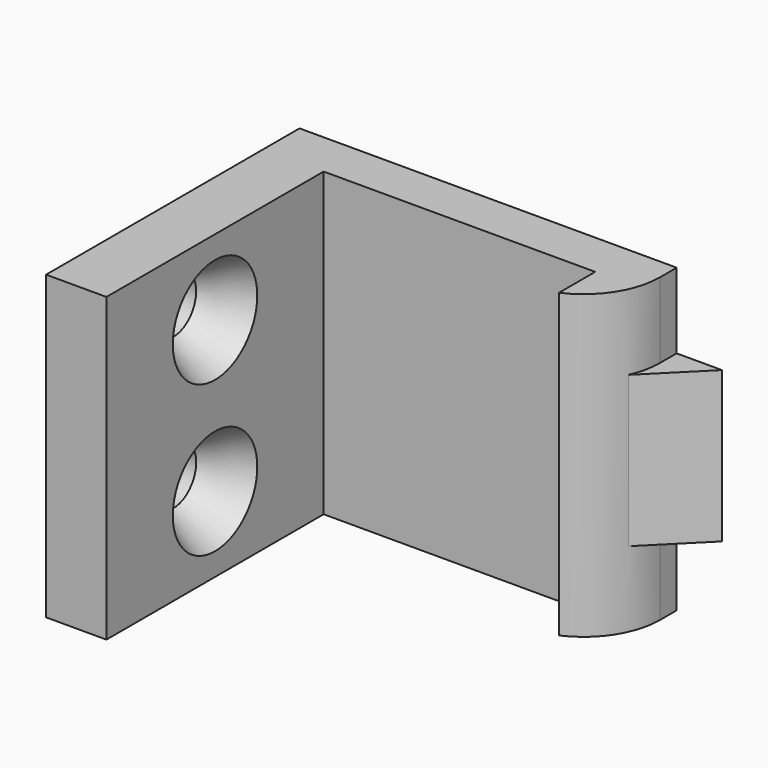
from build123d import *

# Parameters (mm, degrees)
F1_DEPTH       = 20
F2_DEPTH       = 15
F3_DEPTH       = 5
F5_D           = 3.8
F5_DEPTH       = 20
F5_CSINK_D     = 7
F5_CSINK_ANGLE = 60
F5_TIP         = 1.1416351762
F6_T4_DEPTH    = 43.1732604525
F6_T10_DEPTH   = 43.1732604525
F6_T16_DEPTH   = 43.1732604525
F6_T23_DEPTH   = 43.1732604525
F6_T29_DEPTH   = 43.1732604525


# Not quite as in the source:
# - a fillet or chamfer that OpenCascade refuses, or shapes differently, is made with other operations: its cross-section is extruded or revolved along the edge and cut away or added


with BuildPart() as f1:
    # F0 (on Top) → F1 (new body)
    with BuildSketch(Plane.XY):
        Polygon((-23.1947004795, 4.0139819533), (-23.1947004795, -16.9860180467), (-19.1947004795, -16.9860180467), (-19.1947004795, 1.0139819533), (-1.1947004795, 1.0139819533), (-1.1947004795, -1.9860180467), (1.8052995205, -1.9860180467), (1.8052995205, 1.0139819533), (1.8052995205, 4.0139819533), align=None)
    extrude(amount=F1_DEPTH)

    # F0 (on Top) → F2 (join)
    with BuildSketch(Plane.XY):
        Polygon((4.8052995205, 4.0139819533), (1.8052995205, 4.0139819533), (1.8052995205, 1.0139819533), align=None)
    extrude(amount=F2_DEPTH)

    # F0 (on Top) → F3 (cut)
    with BuildSketch(Plane.XY):
        Polygon((4.8052995205, 4.0139819533), (1.8052995205, 4.0139819533), (1.8052995205, 1.0139819533), align=None)
    extrude(amount=F3_DEPTH, mode=Mode.SUBTRACT)

    # F5
    with Locations(Plane.YZ.offset(-19.1947004795)):
        with Locations((-7.9860180467, 15), (-7.9860180467, 5)):
            CounterSinkHole(F5_D / 2, F5_CSINK_D / 2, depth=F5_DEPTH, counter_sink_angle=F5_CSINK_ANGLE)
            with Locations((0, 0, -(F5_DEPTH + F5_TIP / 2))):  # 118° drill point
                Cone(0, F5_D / 2, F5_TIP, mode=Mode.SUBTRACT)

    # F6: fillet of radius 5.08 on 1 edges, made by hand


with BuildPart() as f6_tool2:
    # F6_s3 → F6_t4 (new body)
    with BuildSketch(Plane.XY.offset(-11.5866302263)):
        with BuildLine():
            ThreePointArc((1.8052995205, 2.6486340438), (0.9898510796, -0.1118007046), (-1.1947004795, -1.9860180467))
            Line((-1.1947004795, -1.9860180467), (-1.1531004795, -2.0787110885))
            ThreePointArc((-1.1531004795, -2.0787110885), (0.3052995205, -2.0876180467), (1.8052995205, -2.0876180467))
            Line((1.8052995205, -2.0876180467), (1.9068995205, -1.9860180467))
            Line((1.9068995205, -1.9860180467), (1.9068995205, 2.6486340438))
            Line((1.9068995205, 2.6486340438), (1.8052995205, 2.6486340438))
        make_face()
    extrude(amount=F6_T4_DEPTH)

    split(bisect_by=Plane(origin=(0.3956587836, -0.3956587836, 0), x_dir=(0, 0, 1), z_dir=(-0.7071067812, 0.7071067812, 0)), keep=Keep.TOP)

    split(bisect_by=Plane.XY.offset(5), keep=Keep.BOTTOM)


with BuildPart() as f1_1:
    add(f1.part)

    # F6_t1: cut F6_tool2
    add(f6_tool2.part, mode=Mode.SUBTRACT)


with BuildPart() as f6_tool8:
    # F6_s9 → F6_t10 (new body)
    with BuildSketch(Plane.XY.offset(-11.5866302263)):
        with BuildLine():
            ThreePointArc((1.8052995205, 2.6486340438), (0.9898510796, -0.1118007046), (-1.1947004795, -1.9860180467))
            Line((-1.1947004795, -1.9860180467), (-1.1531004795, -2.0787110885))
            ThreePointArc((-1.1531004795, -2.0787110885), (0.3052995205, -2.0876180467), (1.8052995205, -2.0876180467))
            Line((1.8052995205, -2.0876180467), (1.9068995205, -1.9860180467))
            Line((1.9068995205, -1.9860180467), (1.9068995205, 2.6486340438))
            Line((1.9068995205, 2.6486340438), (1.8052995205, 2.6486340438))
        make_face()
    extrude(amount=F6_T10_DEPTH)

    split(bisect_by=Plane(origin=(0.3956587836, -0.3956587836, 0), x_dir=(0, 0, 1), z_dir=(0.7071067812, -0.7071067812, 0)), keep=Keep.TOP)

    split(bisect_by=Plane.XY.offset(5), keep=Keep.BOTTOM)


with BuildPart() as f1_2:
    add(f1_1.part)

    # F6_t7: cut F6_tool8
    add(f6_tool8.part, mode=Mode.SUBTRACT)


with BuildPart() as f6_tool14:
    # F6_s15 → F6_t16 (new body)
    with BuildSketch(Plane.XY.offset(-11.5866302263)):
        with BuildLine():
            ThreePointArc((1.8052995205, 2.6486340438), (0.9898510796, -0.1118007046), (-1.1947004795, -1.9860180467))
            Line((-1.1947004795, -1.9860180467), (-1.1531004795, -2.0787110885))
            ThreePointArc((-1.1531004795, -2.0787110885), (0.3052995205, -2.0876180467), (1.8052995205, -2.0876180467))
            Line((1.8052995205, -2.0876180467), (1.9068995205, -1.9860180467))
            Line((1.9068995205, -1.9860180467), (1.9068995205, 2.6486340438))
            Line((1.9068995205, 2.6486340438), (1.8052995205, 2.6486340438))
        make_face()
    extrude(amount=F6_T16_DEPTH)

    split(bisect_by=Plane.XY.offset(15), keep=Keep.BOTTOM)

    split(bisect_by=Plane(origin=(0.3956587836, -0.3956587836, 0), x_dir=(0, 0, 1), z_dir=(0.7071067812, -0.7071067812, 0)), keep=Keep.TOP)

    split(bisect_by=Plane.XY.offset(5), keep=Keep.TOP)


with BuildPart() as f1_3:
    add(f1_2.part)

    # F6_t13: cut F6_tool14
    add(f6_tool14.part, mode=Mode.SUBTRACT)


with BuildPart() as f6_tool21:
    # F6_s22 → F6_t23 (new body)
    with BuildSketch(Plane.XY.offset(-11.5866302263)):
        with BuildLine():
            ThreePointArc((1.8052995205, 2.6486340438), (0.9898510796, -0.1118007046), (-1.1947004795, -1.9860180467))
            Line((-1.1947004795, -1.9860180467), (-1.1531004795, -2.0787110885))
            ThreePointArc((-1.1531004795, -2.0787110885), (0.3052995205, -2.0876180467), (1.8052995205, -2.0876180467))
            Line((1.8052995205, -2.0876180467), (1.9068995205, -1.9860180467))
            Line((1.9068995205, -1.9860180467), (1.9068995205, 2.6486340438))
            Line((1.9068995205, 2.6486340438), (1.8052995205, 2.6486340438))
        make_face()
    extrude(amount=F6_T23_DEPTH)

    split(bisect_by=Plane.XY.offset(15), keep=Keep.TOP)

    split(bisect_by=Plane(origin=(0.3956587836, -0.3956587836, 0), x_dir=(0, 0, 1), z_dir=(-0.7071067812, 0.7071067812, 0)), keep=Keep.TOP)


with BuildPart() as f1_4:
    add(f1_3.part)

    # F6_t20: cut F6_tool21
    add(f6_tool21.part, mode=Mode.SUBTRACT)


with BuildPart() as f6_tool27:
    # F6_s28 → F6_t29 (new body)
    with BuildSketch(Plane.XY.offset(-11.5866302263)):
        with BuildLine():
            ThreePointArc((1.8052995205, 2.6486340438), (0.9898510796, -0.1118007046), (-1.1947004795, -1.9860180467))
            Line((-1.1947004795, -1.9860180467), (-1.1531004795, -2.0787110885))
            ThreePointArc((-1.1531004795, -2.0787110885), (0.3052995205, -2.0876180467), (1.8052995205, -2.0876180467))
            Line((1.8052995205, -2.0876180467), (1.9068995205, -1.9860180467))
            Line((1.9068995205, -1.9860180467), (1.9068995205, 2.6486340438))
            Line((1.9068995205, 2.6486340438), (1.8052995205, 2.6486340438))
        make_face()
    extrude(amount=F6_T29_DEPTH)

    split(bisect_by=Plane.XY.offset(15), keep=Keep.TOP)

    split(bisect_by=Plane(origin=(0.3956587836, -0.3956587836, 0), x_dir=(0, 0, 1), z_dir=(0.7071067812, -0.7071067812, 0)), keep=Keep.TOP)


with BuildPart() as f1_5:
    add(f1_4.part)

    # F6_t26: cut F6_tool27
    add(f6_tool27.part, mode=Mode.SUBTRACT)


solid = f1_5.part
